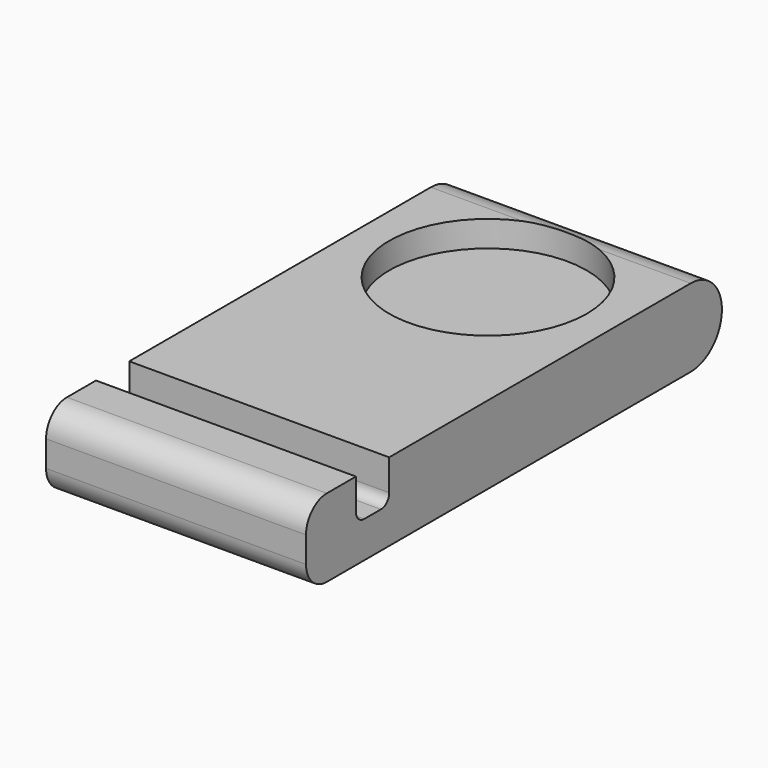
from build123d import *

# Parameters (mm, degrees)
F0_W        = 12.7
F0_H        = 25.4
F1_DEPTH    = 3.81
F2_R        = 4.826
F3_DEPTH    = 1.27
F4_W        = 2.032
F4_H        = 2.032
F5_DEPTH    = 25.4
F6_R        = 0.508
F7_T1_DEPTH = 22.225
F8_R        = 1.27


# Not quite as in the source:
# - a fillet or chamfer that OpenCascade refuses, or shapes differently, is made with other operations: its cross-section is extruded or revolved along the edge and cut away or added


with BuildPart() as f1:
    # F0 (on Top) → F1 (new body)
    with BuildSketch(Plane.XY):
        with Locations((6.35, -12.7)):
            Rectangle(F0_W, F0_H)
    extrude(amount=F1_DEPTH)

    # F2 (on face) → F3 (cut)
    with BuildSketch(Plane.XY.offset(3.81)):
        with Locations((6.35, -6.35)):
            Circle(F2_R)
    extrude(amount=-F3_DEPTH, mode=Mode.SUBTRACT)

    # F4 (on face) → F5 (cut)
    with BuildSketch(Plane.YZ.offset(12.7)):
        with Locations((-21.336, 2.794)):
            Rectangle(F4_W, F4_H)
    extrude(amount=-F5_DEPTH, mode=Mode.SUBTRACT)

    # F6
    f6_edges = [f1.edges().sort_by_distance(p)[0] for p in [
        (6.35, -20.32, 1.778),
        (6.35, -22.352, 1.778),
    ]]
    fillet(f6_edges, radius=F6_R)

    # F7: fillet of radius 1.905 on 2 edges, made by hand

    # F7_s2 → F7_t1 (cut)
    with BuildSketch(Plane.YZ.offset(-4.7625)):
        with BuildLine():
            ThreePointArc((0, 1.905), (-0.5579615818, 0.5579615818), (-1.905, 0))
            Line((-1.905, 0), (0, 0))
            Line((0, 0), (0, 1.905))
        make_face()
        with BuildLine():
            ThreePointArc((-1.905, 3.81), (-0.5579615818, 3.2520384182), (0, 1.905))
            Line((0, 1.905), (0, 3.81))
            Line((0, 3.81), (-1.905, 3.81))
        make_face()
    extrude(amount=F7_T1_DEPTH, mode=Mode.SUBTRACT)

    # F8
    f8_edges = [f1.edges().sort_by_distance(p)[0] for p in [
        (6.35, -25.4, 3.81),
        (6.35, -25.4, 0),
    ]]
    fillet(f8_edges, radius=F8_R)


solid = f1.part
